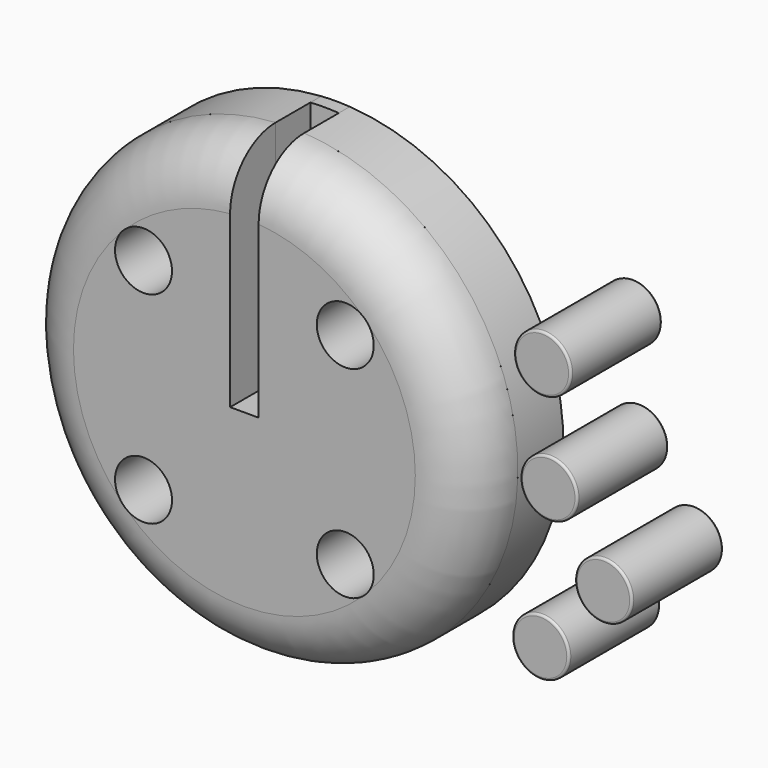
from build123d import *

# Parameters (mm, degrees)
F0_R        = 6.35
F0_W        = 6.35
F0_H        = 50.700684167
F1_DEPTH    = 12.7
F2_DEPTH    = 12.7
F4_START    = 3.048
F4_DEPTH    = 22.352
F5_T4_DEPTH = 6.35
F6_R        = 6.35
F7_DEPTH    = 25.4
F8_R        = 0.508
F8_2_R      = 0.508
F8_3_R      = 0.508
F8_4_R      = 0.508


# Not quite as in the source:
# - a fillet or chamfer that OpenCascade refuses, or shapes differently, is made with other operations: its cross-section is extruded or revolved along the edge and cut away or added


with BuildPart() as f1:
    # F0 (on Front) → F1 (new body)
    with BuildSketch(Plane.XZ):
        with BuildLine():
            ThreePointArc((-14.3502756187, 59.6704592896), (-45.9556580202, -28.0567694096), (39.6247243813, 8.9697751226))
            ThreePointArc((39.6247243813, 8.9697751226), (25.8512689136, 43.7501575242), (-8.0002756187, 59.6704592896))
            Line((-8.0002756187, 59.6704592896), (-8.0002756187, 8.9697751226))
            Line((-8.0002756187, 8.9697751226), (-14.3502756187, 8.9697751226))
            Line((-14.3502756187, 8.9697751226), (-14.3502756187, 59.6704592896))
        make_face()
        with Locations((-33.6597404378, -13.5146896965)):
            Circle(F0_R, mode=Mode.SUBTRACT)
        with Locations((11.3091892005, -13.5146896965)):
            Circle(F0_R, mode=Mode.SUBTRACT)
        with Locations((-33.6597404378, 31.4542399417)):
            Circle(F0_R, mode=Mode.SUBTRACT)
        with Locations((11.3091892005, 31.4542399417)):
            Circle(F0_R, mode=Mode.SUBTRACT)
        with BuildLine():
            Line((-14.3502756187, 59.6704592896), (-8.0002756187, 59.6704592896))
            ThreePointArc((-8.0002756187, 59.6704592896), (-11.1752756187, 59.7697751226), (-14.3502756187, 59.6704592896))
        make_face()
        with Locations((-11.1752756187, 34.3201172061)):
            Rectangle(F0_W, F0_H)
    extrude(amount=F1_DEPTH)


with BuildPart() as f2:
    # F2 (new): a face of the model
    f2_faces = [f1.part.faces().sort_by_distance(p)[0] for p in [
        (-11.1752756187, -12.7, 8.9697751226),
    ]]
    extrude(f2_faces, amount=F2_DEPTH)

    # F3: fillet of radius 12.7 on 1 edges, made by hand

    # F3_s1 → F3_t2 (revolve, cut)
    with BuildSketch(Plane(origin=(-11.6911371288, 0, 0.732127406), x_dir=(0, 1, 0), z_dir=(0.9980449639, 0, -0.0625))):
        with BuildLine():
            ThreePointArc((-12.7, 59.0537841624), (-21.6802561211, 55.3340402835), (-25.4, 46.3537841624))
            Line((-25.4, 46.3537841624), (-25.4, 59.0537841624))
            Line((-25.4, 59.0537841624), (-12.7, 59.0537841624))
        make_face()
    revolve(axis=Axis((-11.1752756187, -25.4, 8.9697751226), (0, -1, 0)), mode=Mode.SUBTRACT)


with BuildPart() as f4_tool:
    # F0 (on Front) → F4 (new body)
    with BuildSketch(Plane.XZ.offset(F4_START)):
        with BuildLine():
            Line((-14.3502756187, 59.6704592896), (-8.0002756187, 59.6704592896))
            ThreePointArc((-8.0002756187, 59.6704592896), (-11.1752756187, 59.7697751226), (-14.3502756187, 59.6704592896))
        make_face()
        with Locations((-11.1752756187, 34.3201172061)):
            Rectangle(F0_W, F0_H)
    extrude(amount=F4_DEPTH)


with BuildPart() as f1_1:
    add(f1.part)

    # F4: cut by f4_tool
    add(f4_tool.part, mode=Mode.SUBTRACT)

    # F5: chamfer of 19.05 on 1 edges, made by hand


with BuildPart() as f2_1:
    add(f2.part)

    # F4: cut by f4_tool
    add(f4_tool.part, mode=Mode.SUBTRACT)


with BuildPart() as f5_tool2:
    # F5_s3 → F5_t4 (new body)
    with BuildSketch(Plane.YZ.offset(-8.0002756187)):
        Polygon((-12.7, -10.0802248774), (6.35, 8.9697751226), (-12.7, 8.9697751226), align=None)
    extrude(amount=-F5_T4_DEPTH)

    split(bisect_by=Plane.XZ.offset(3.048), keep=Keep.TOP)


with BuildPart() as f1_2:
    add(f1_1.part)

    # F5_t1: cut F5_tool2
    add(f5_tool2.part, mode=Mode.SUBTRACT)


with BuildPart() as f7:
    # F6 (on Front) → F7 (new body)
    with BuildSketch(Plane.XZ):
        with Locations((55.2439391613, 40.0804132223)):
            Circle(F6_R)
    extrude(amount=F7_DEPTH)

    # F8
    f8_edges = [f7.edges().sort_by_distance(p)[0] for p in [
        (48.893939, -25.4, 40.080413),
        (48.893939, 0, 40.080413),
    ]]
    fillet(f8_edges, radius=F8_R)


with BuildPart() as f7b:
    # F6 (on Front) → F7, piece 2 (new body)
    with BuildSketch(Plane.XZ):
        with Locations((56.6665492952, 16.0992704332)):
            Circle(F6_R)
    extrude(amount=F7_DEPTH)

    # F8#2
    f8_2_edges = [f7b.edges().sort_by_distance(p)[0] for p in [
        (50.316549, -25.4, 16.09927),
        (50.316549, 0, 16.09927),
    ]]
    fillet(f8_2_edges, radius=F8_2_R)


with BuildPart() as f7c:
    # F6 (on Front) → F7, piece 3 (new body)
    with BuildSketch(Plane.XZ):
        with Locations((54.8374764621, -15.6046124175)):
            Circle(F6_R)
    extrude(amount=F7_DEPTH)

    # F8#3
    f8_3_edges = [f7c.edges().sort_by_distance(p)[0] for p in [
        (48.487476, 0, -15.604612),
        (48.487476, -25.4, -15.604612),
    ]]
    fillet(f8_3_edges, radius=F8_3_R)


with BuildPart() as f7d:
    # F6 (on Front) → F7, piece 4 (new body)
    with BuildSketch(Plane.XZ):
        with Locations((68.8603520393, 0)):
            Circle(F6_R)
    extrude(amount=F7_DEPTH)

    # F8#4
    f8_4_edges = [f7d.edges().sort_by_distance(p)[0] for p in [
        (62.510352, -25.4, 0),
        (62.510352, 0, 0),
    ]]
    fillet(f8_4_edges, radius=F8_4_R)


solid = Compound([f2_1.part, f1_2.part, f7.part, f7b.part, f7c.part, f7d.part])
